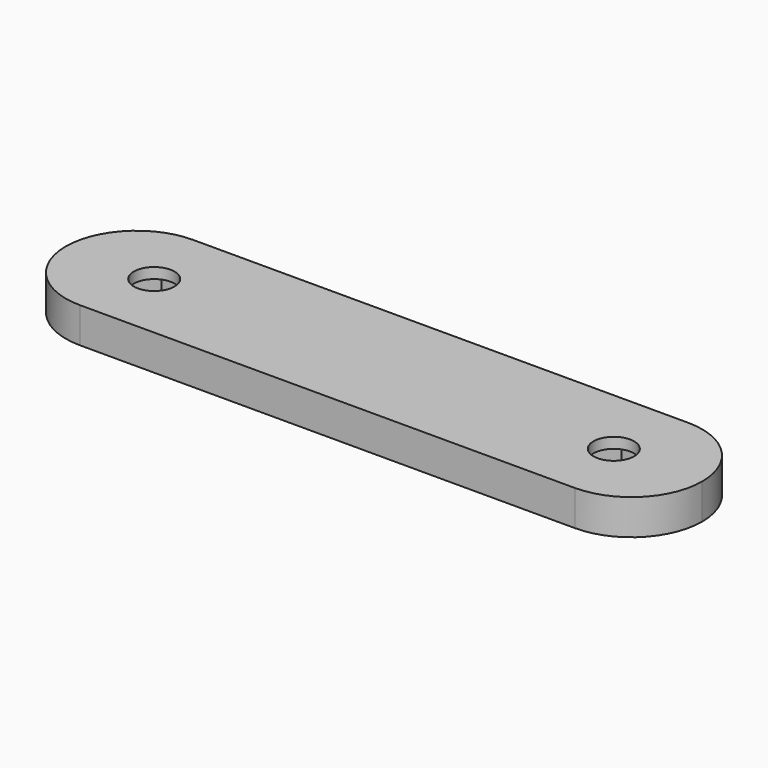
from build123d import *

# Parameters (mm, degrees)
F1_W     = 36
F1_H     = 8
F3_DEPTH = 2
F0_R     = 1.15
F4_DEPTH = 2.001
F5_DEPTH = 1.4
F6_R     = 3.99999


# Not quite as in the source:
# - a fillet or chamfer is up to 0.001 mm smaller than in the source, because OpenCascade refuses the exact size


with BuildPart() as f3:
    # F1 (on Top) → F3 (new body)
    with BuildSketch(Plane.XY):
        Rectangle(F1_W, F1_H)
    extrude(amount=F3_DEPTH)

    # F0 (on Top) → F4 (cut, through all)
    with BuildSketch(Plane.XY):
        with Locations((-13, 0)):
            Circle(F0_R)
        with Locations((13, 0)):
            Circle(F0_R)
    extrude(amount=F4_DEPTH, mode=Mode.SUBTRACT)

    # F2 (on Top) → F5 (cut)
    with BuildSketch(Plane.XY):
        Polygon((-11.8943742345, -1.915), (-10.788748469, 0), (-11.8943742345, 1.915), (-13, 1.915), (-14.1056257655, 1.915), (-15.211251531, 0), (-14.1056257655, -1.915), (-13, -1.915), align=None)
        Polygon((14.1056257655, -1.915), (15.211251531, 0), (14.1056257655, 1.915), (13, 1.915), (11.8943742345, 1.915), (10.788748469, 0), (11.8943742345, -1.915), (13, -1.915), align=None)
    extrude(amount=F5_DEPTH, mode=Mode.SUBTRACT)

    # F6 (radius 4 in the source; OpenCascade refuses exactly that, so slightly less here)
    f6_edges = [f3.edges().sort_by_distance(p)[0] for p in [
        (-18, 4, 1),
        (-18, -4, 1),
        (18, -4, 1),
        (18, 4, 1),
    ]]
    fillet(f6_edges, radius=F6_R)


solid = f3.part
